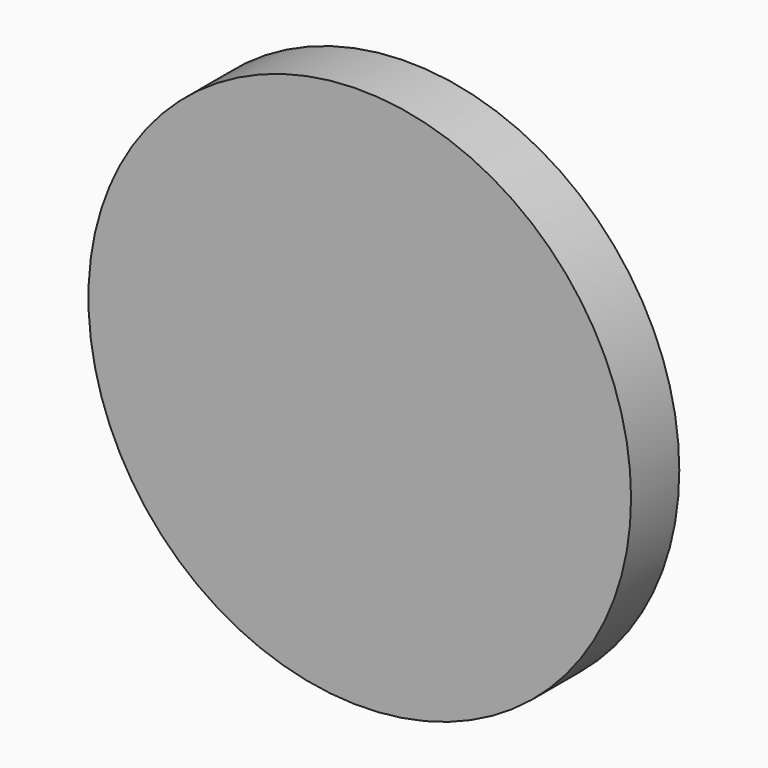
from build123d import *

# Parameters (mm, degrees)
F0_R     = 112.5
F5_DEPTH = 12.5


# Not quite as in the source:
# - the program builds the solid bodies; features that only make, move or delete a surface that nothing else refers to are left out


with BuildPart() as f5:
    # F0 (on Front) → F5 (new body, symmetric)
    with BuildSketch(Plane.XZ):
        Circle(F0_R)
    extrude(amount=F5_DEPTH, both=True)


solid = f5.part
